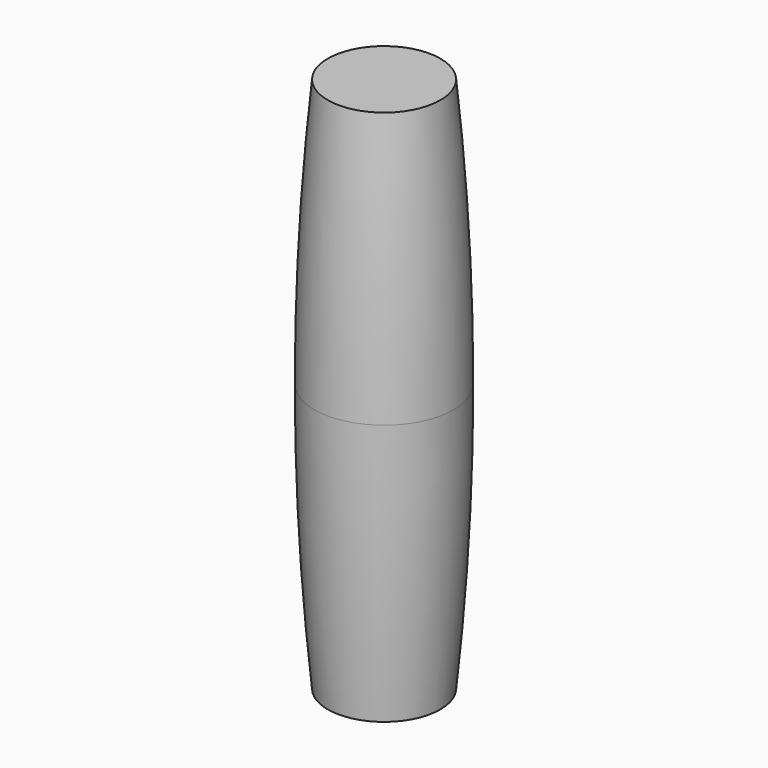
from build123d import *


# Not quite as in the source:
# - a feature names something its author has since deleted; it is built from what else it names


with BuildPart() as f1:
    # F0 (on Front) → F1 (revolve)
    with BuildSketch(Plane.XZ):
        with BuildLine():
            Line((0, 100), (0, 0))
            Line((0, 0), (0, -100))
            Line((0, -100), (20.9873259794, -100))
            ThreePointArc((20.9873259794, -100), (24.7459899382, -50.0633286095), (25.9999999976, -0.0011056954))
            Line((26, -0.0011056954), (26, 0))
            ThreePointArc((25.9999999994, 0), (25.9999999986, 0.0005528477), (25.9999999976, 0.0011056954))
            ThreePointArc((25.9999999976, 0.0011056954), (24.7459899382, 50.0633286095), (20.9873259794, 100))
            Line((20.9873259794, 100), (0, 100))
        make_face()
    revolve(axis=Axis((0, 0, 50), (0, 0, 1)))


solid = f1.part
